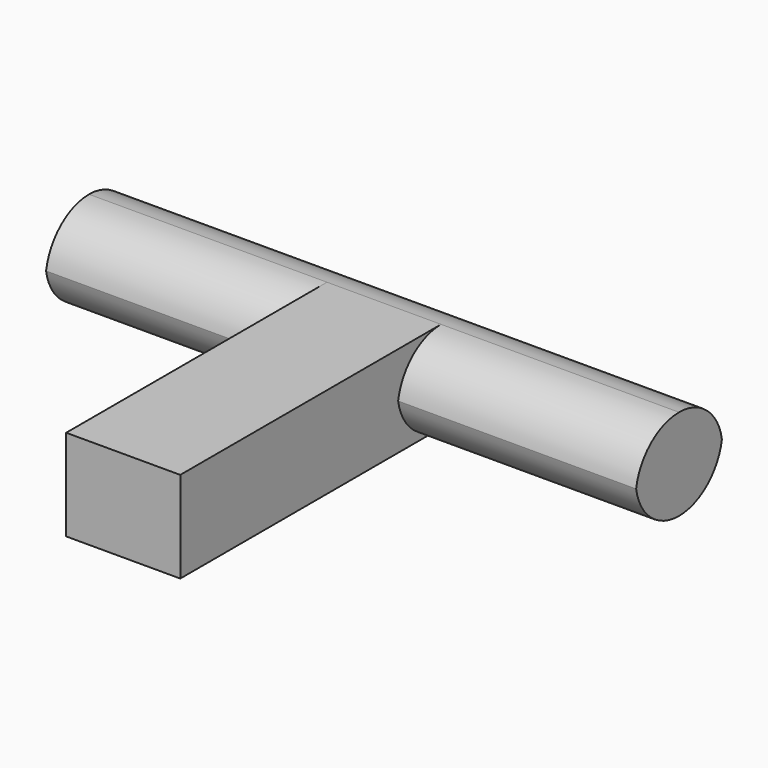
from build123d import *

# Parameters (mm, degrees)
F0_W         = 10.668002069
F0_H         = 8.5344007239
F1_DEPTH     = 25.4
F2_W         = 22.2503971308
F2_H         = 8.5344007239
F2_W_2       = 10.668002069
F3_DEPTH     = 10.16
F4_T1_DEPTH  = 80.5687963307
F4_T3_DEPTH  = 34.9503971308
F4_T5_DEPTH  = 34.9503971308
F4_T10_DEPTH = 47.6503971308
F4_T15_DEPTH = 47.6503971308
F4_T20_DEPTH = 47.6503971308
F4_T25_DEPTH = 47.6503971308


# Not quite as in the source:
# - a fillet or chamfer that OpenCascade refuses, or shapes differently, is made with other operations: its cross-section is extruded or revolved along the edge and cut away or added


with BuildPart() as f1:
    # F0 (on Front) → F1 (new body)
    with BuildSketch(Plane.XZ):
        Rectangle(F0_W, F0_H)
    extrude(amount=F1_DEPTH)

    # F2 (on face) → F3 (join)
    with BuildSketch(Plane(origin=(0, 0, 0), x_dir=(-1, 0, 0), z_dir=(0, 1, 0))):
        with Locations((-16.4591995999, 0)):
            Rectangle(F2_W, F2_H)
        Rectangle(F2_W_2, F2_H)
        with Locations((16.4591995999, 0)):
            Rectangle(F2_W, F2_H)
    extrude(amount=F3_DEPTH)

    # F4: fillet of radius 5.08 on 6 edges, made by hand

    # F4_s2 → F4_t1 (cut)
    with BuildSketch(Plane.YZ.offset(-40.2843981653)):
        with BuildLine():
            ThreePointArc((10.16, -0.8127996381), (8.6721024484, 2.7793028104), (5.08, 4.2672003619))
            Line((5.08, 4.2672003619), (10.16, 4.2672003619))
            Line((10.16, 4.2672003619), (10.16, -0.8127996381))
        make_face()
        with BuildLine():
            ThreePointArc((5.08, -4.2672003619), (8.6721024484, -2.7793028104), (10.16, 0.8127996381))
            Line((10.16, 0.8127996381), (10.16, -4.2672003619))
            Line((10.16, -4.2672003619), (5.08, -4.2672003619))
        make_face()
    extrude(amount=F4_T1_DEPTH, mode=Mode.SUBTRACT)

    # F4_s4 → F4_t3 (cut)
    with BuildSketch(Plane.YZ.offset(5.3340010345)):
        with BuildLine():
            ThreePointArc((0, -0.8127996381), (1.4878975516, 2.7793028104), (5.08, 4.2672003619))
            Line((5.08, 4.2672003619), (0, 4.2672003619))
            Line((0, 4.2672003619), (0, -0.8127996381))
        make_face()
        with BuildLine():
            ThreePointArc((5.08, -4.2672003619), (1.4878975516, -2.7793028104), (0, 0.8127996381))
            Line((0, 0.8127996381), (0, -4.2672003619))
            Line((0, -4.2672003619), (5.08, -4.2672003619))
        make_face()
    extrude(amount=F4_T3_DEPTH, mode=Mode.SUBTRACT)

    # F4_s6 → F4_t5 (cut)
    with BuildSketch(Plane.YZ.offset(-40.2843981653)):
        with BuildLine():
            ThreePointArc((5.08, -4.2672003619), (1.4878975516, -2.7793028104), (0, 0.8127996381))
            Line((0, 0.8127996381), (0, -4.2672003619))
            Line((0, -4.2672003619), (5.08, -4.2672003619))
        make_face()
        with BuildLine():
            ThreePointArc((0, -0.8127996381), (1.4878975516, 2.7793028104), (5.08, 4.2672003619))
            Line((5.08, 4.2672003619), (0, 4.2672003619))
            Line((0, 4.2672003619), (0, -0.8127996381))
        make_face()
    extrude(amount=F4_T5_DEPTH, mode=Mode.SUBTRACT)


with BuildPart() as f4_tool8:
    # F4_s9 → F4_t10 (new body)
    with BuildSketch(Plane.YZ.offset(-7.3659989655)):
        with BuildLine():
            ThreePointArc((0, -0.8127996381), (1.4878975516, 2.7793028104), (5.08, 4.2672003619))
            Line((5.08, 4.2672003619), (0, 4.2672003619))
            Line((0, 4.2672003619), (0, -0.8127996381))
        make_face()
    extrude(amount=F4_T10_DEPTH)

    split(bisect_by=Plane.YZ.offset(-5.3340010345), keep=Keep.BOTTOM)


with BuildPart() as f1_1:
    add(f1.part)

    # F4_t7: cut F4_tool8
    add(f4_tool8.part, mode=Mode.SUBTRACT)


with BuildPart() as f4_tool13:
    # F4_s14 → F4_t15 (new body)
    with BuildSketch(Plane.YZ.offset(40.2843981653)):
        with BuildLine():
            ThreePointArc((5.08, -4.2672003619), (1.4878975516, -2.7793028104), (0, 0.8127996381))
            Line((0, 0.8127996381), (0, -4.2672003619))
            Line((0, -4.2672003619), (5.08, -4.2672003619))
        make_face()
    extrude(amount=-F4_T15_DEPTH)

    split(bisect_by=Plane.YZ.offset(-5.3340010345), keep=Keep.BOTTOM)


with BuildPart() as f1_2:
    add(f1_1.part)

    # F4_t12: cut F4_tool13
    add(f4_tool13.part, mode=Mode.SUBTRACT)


with BuildPart() as f4_tool18:
    # F4_s19 → F4_t20 (new body)
    with BuildSketch(Plane.YZ.offset(7.3659989655)):
        with BuildLine():
            ThreePointArc((5.08, -4.2672003619), (1.4878975516, -2.7793028104), (0, 0.8127996381))
            Line((0, 0.8127996381), (0, -4.2672003619))
            Line((0, -4.2672003619), (5.08, -4.2672003619))
        make_face()
    extrude(amount=-F4_T20_DEPTH)

    split(bisect_by=Plane.YZ.offset(5.3340010345), keep=Keep.TOP)


with BuildPart() as f1_3:
    add(f1_2.part)

    # F4_t17: cut F4_tool18
    add(f4_tool18.part, mode=Mode.SUBTRACT)


with BuildPart() as f4_tool23:
    # F4_s24 → F4_t25 (new body)
    with BuildSketch(Plane.YZ.offset(-40.2843981653)):
        with BuildLine():
            ThreePointArc((0, -0.8127996381), (1.4878975516, 2.7793028104), (5.08, 4.2672003619))
            Line((5.08, 4.2672003619), (0, 4.2672003619))
            Line((0, 4.2672003619), (0, -0.8127996381))
        make_face()
    extrude(amount=F4_T25_DEPTH)

    split(bisect_by=Plane.YZ.offset(5.3340010345), keep=Keep.TOP)


with BuildPart() as f1_4:
    add(f1_3.part)

    # F4_t22: cut F4_tool23
    add(f4_tool23.part, mode=Mode.SUBTRACT)


solid = f1_4.part
